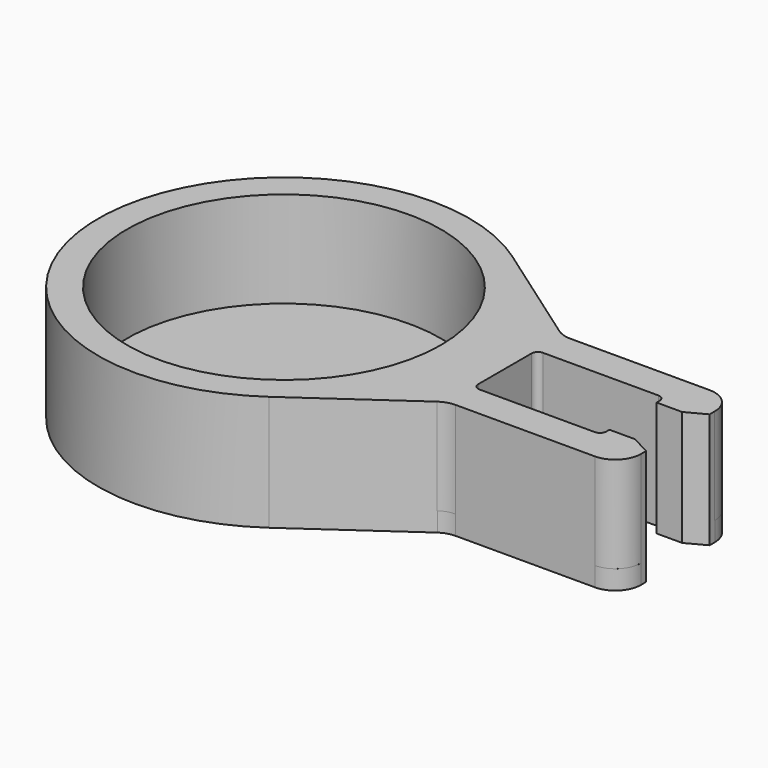
from build123d import *

# Parameters (mm, degrees)
F0_R        = 31.115
F1_DEPTH    = 19.05
F2_R        = 1.27
F3_R        = 5.08
F4_DEPTH    = 3.81
F5_T1_DEPTH = 6.9847500098
F6_T1_DEPTH = 7.826096392
F6_T3_DEPTH = 29.2095000049


# Not quite as in the source:
# - a fillet or chamfer that OpenCascade refuses, or shapes differently, is made with other operations: its cross-section is extruded or revolved along the edge and cut away or added


with BuildPart() as f1:
    # F0 (on Top) → F1 (new body)
    with BuildSketch(Plane.XY):
        with BuildLine():
            ThreePointArc((-22.6388816051, -22.2593853014), (-11.1319360334, -9.104404806), (-6.985, 7.874))
            ThreePointArc((-6.985, 7.874), (-11.1319360334, 24.852404806), (-22.6388816051, 38.0073853014))
            ThreePointArc((-22.6388816051, 38.0073853014), (-80.645, 7.874), (-22.6388816051, -22.2593853014))
        make_face()
        with Locations((-43.815, 7.874)):
            Circle(F0_R, mode=Mode.SUBTRACT)
        with BuildLine():
            Line((-6.985, 7.874), (0, 7.874))
            Line((0, 7.874), (0, 15.748))
            Line((0, 15.748), (25.4, 15.748))
            Line((25.4, 15.748), (34.29, 15.748))
            Line((34.29, 15.748), (34.29, 22.098))
            Line((34.29, 22.098), (0, 22.098))
            Line((0, 22.098), (-22.6388816051, 38.0073853014))
            ThreePointArc((-22.6388816051, 38.0073853014), (-11.1319360334, 24.852404806), (-6.985, 7.874))
        make_face()
        with BuildLine():
            Line((25.4, 0), (0, 0))
            Line((0, 0), (0, 7.874))
            Line((0, 7.874), (-6.985, 7.874))
            ThreePointArc((-6.985, 7.874), (-11.1319360334, -9.104404806), (-22.6388816051, -22.2593853014))
            Line((-22.6388816051, -22.2593853014), (0, -6.35))
            Line((0, -6.35), (34.29, -6.35))
            Line((34.29, -6.35), (34.29, 0))
            Line((34.29, 0), (25.4, 0))
        make_face()
        Polygon((25.4, 2.032), (25.4, 0), (34.29, 0), (30.48, 2.032), align=None)
        Polygon((34.29, 15.748), (25.4, 15.748), (25.4, 13.716), (30.48, 13.716), align=None)
    extrude(amount=F1_DEPTH)

    # F2
    f2_edges = [f1.edges().sort_by_distance(p)[0] for p in [
        (0, 15.748, 9.525),
        (25.4, 15.748, 9.525),
        (0, 0, 9.525),
        (25.4, 0, 9.525),
    ]]
    fillet(f2_edges, radius=F2_R)

    # F3
    f3_edges = [f1.edges().sort_by_distance(p)[0] for p in [
        (34.29, -6.35, 9.525),
        (34.29, 22.098, 9.525),
        (0, -6.35, 9.525),
        (0, 22.098, 9.525),
    ]]
    fillet(f3_edges, radius=F3_R)

    # F0 (on Top) → F4 (join)
    with BuildSketch(Plane.XY):
        with BuildLine():
            ThreePointArc((-22.6388816051, -22.2593853014), (-11.1319360334, -9.104404806), (-6.985, 7.874))
            ThreePointArc((-6.985, 7.874), (-11.1319360334, 24.852404806), (-22.6388816051, 38.0073853014))
            ThreePointArc((-22.6388816051, 38.0073853014), (-80.645, 7.874), (-22.6388816051, -22.2593853014))
        make_face()
        with Locations((-43.815, 7.874)):
            Circle(F0_R, mode=Mode.SUBTRACT)
        with Locations((-43.815, 7.874)):
            Circle(F0_R)
        with BuildLine():
            Line((25.4, 0), (0, 0))
            Line((0, 0), (0, 7.874))
            Line((0, 7.874), (-6.985, 7.874))
            ThreePointArc((-6.985, 7.874), (-11.1319360334, -9.104404806), (-22.6388816051, -22.2593853014))
            Line((-22.6388816051, -22.2593853014), (0, -6.35))
            Line((0, -6.35), (34.29, -6.35))
            Line((34.29, -6.35), (34.29, 0))
            Line((34.29, 0), (25.4, 0))
        make_face()
        with BuildLine():
            Line((-6.985, 7.874), (0, 7.874))
            Line((0, 7.874), (0, 15.748))
            Line((0, 15.748), (25.4, 15.748))
            Line((25.4, 15.748), (34.29, 15.748))
            Line((34.29, 15.748), (34.29, 22.098))
            Line((34.29, 22.098), (0, 22.098))
            Line((0, 22.098), (-22.6388816051, 38.0073853014))
            ThreePointArc((-22.6388816051, 38.0073853014), (-11.1319360334, 24.852404806), (-6.985, 7.874))
        make_face()
        Polygon((34.29, 15.748), (25.4, 15.748), (25.4, 13.716), (30.48, 13.716), align=None)
        Polygon((25.4, 2.032), (25.4, 0), (34.29, 0), (30.48, 2.032), align=None)
    extrude(amount=-F4_DEPTH)

    # F5: fillet of radius 1.27 on 4 edges, made by hand

    # F5_s2 → F5_t1 (join)
    with BuildSketch(Plane.XY.offset(-3.81)):
        with BuildLine():
            ThreePointArc((24.1301, -0.0001), (25.0281256121, 0.3718743879), (25.4001, 1.2699))
            Line((25.4001, 1.2699), (25.4255, 1.2699))
            ThreePointArc((25.4255, 1.2699), (25.4254, 0.63495), (25.4254, 0))
            Line((25.4254, 0), (25.4, -0.0254))
            ThreePointArc((25.4, -0.0254), (24.76505, -0.0254), (24.1301, -0.0255))
            Line((24.1301, -0.0255), (24.1301, -0.0001))
        make_face()
        with BuildLine():
            ThreePointArc((25.4001, 14.4781), (25.0281256121, 15.3761256121), (24.1301, 15.7481))
            Line((24.1301, 15.7481), (24.1301, 15.7735))
            ThreePointArc((24.1301, 15.7735), (24.76505, 15.7734), (25.4, 15.7734))
            Line((25.4, 15.7734), (25.4254, 15.748))
            ThreePointArc((25.4254, 15.748), (25.4254, 15.11305), (25.4255, 14.4781))
            Line((25.4255, 14.4781), (25.4001, 14.4781))
        make_face()
        with BuildLine():
            ThreePointArc((1.2699, 15.7481), (0.3718743879, 15.3761256121), (-0.0001, 14.4781))
            Line((-0.0001, 14.4781), (-0.0255, 14.4781))
            ThreePointArc((-0.0255, 14.4781), (-0.0254, 15.11305), (-0.0254, 15.748))
            Line((-0.0254, 15.748), (0, 15.7734))
            ThreePointArc((0, 15.7734), (0.63495, 15.7734), (1.2699, 15.7735))
            Line((1.2699, 15.7735), (1.2699, 15.7481))
        make_face()
        with BuildLine():
            ThreePointArc((-0.0001, 1.2699), (0.3718743879, 0.3718743879), (1.2699, -0.0001))
            Line((1.2699, -0.0001), (1.2699, -0.0255))
            ThreePointArc((1.2699, -0.0255), (0.63495, -0.0254), (0, -0.0254))
            Line((0, -0.0254), (-0.0254, 0))
            ThreePointArc((-0.0254, 0), (-0.0254, 0.63495), (-0.0255, 1.2699))
            Line((-0.0255, 1.2699), (-0.0001, 1.2699))
        make_face()
    extrude(amount=F5_T1_DEPTH)

    # F6: fillet of radius 5.08 on 4 edges, made by hand

    # F6_s2 → F6_t1 (join)
    with BuildSketch(Plane.XY.offset(-3.81)):
        with BuildLine():
            ThreePointArc((-1.3144053628, -7.2735709929), (0.0747322104, -6.5863191265), (1.6064385537, -6.3499))
            Line((1.6064385537, -6.3499), (1.6064385537, -6.2483))
            ThreePointArc((1.6064385537, -6.2483), (0.8032192768, -6.2484), (0, -6.2484))
            Line((0, -6.2484), (-0.0584168783, -6.2668734199))
            ThreePointArc((-0.0584168783, -6.2668734199), (-0.7155908113, -6.7286998251), (-1.3728222412, -7.1904444128))
            Line((-1.3728222412, -7.1904444128), (-1.3144053628, -7.2735709929))
        make_face()
        with BuildLine():
            ThreePointArc((-1.3144053628, 23.0215709929), (0.0747322104, 22.3343191265), (1.6064385537, 22.0979))
            Line((1.6064385537, 22.0979), (1.6064385537, 21.9963))
            ThreePointArc((1.6064385537, 21.9963), (0.8032192768, 21.9964), (0, 21.9964))
            Line((0, 21.9964), (-0.0584168783, 22.0148734199))
            ThreePointArc((-0.0584168783, 22.0148734199), (-0.7155908113, 22.4766998251), (-1.3728222412, 22.9384444128))
            Line((-1.3728222412, 22.9384444128), (-1.3144053628, 23.0215709929))
        make_face()
    extrude(amount=F6_T1_DEPTH)

    # F6_s4 → F6_t3 (cut)
    with BuildSketch(Plane.XY.offset(-16.5097500025)):
        with BuildLine():
            ThreePointArc((29.2101, -6.3501), (32.8022024484, -4.8622024484), (34.2901, -1.2701))
            Line((34.2901, -1.2701), (34.3917, -1.2701))
            ThreePointArc((34.3917, -1.2701), (34.3916, -3.81005), (34.3916, -6.35))
            Line((34.3916, -6.35), (34.29, -6.4516))
            ThreePointArc((34.29, -6.4516), (31.75005, -6.4516), (29.2101, -6.4517))
            Line((29.2101, -6.4517), (29.2101, -6.3501))
        make_face()
        with BuildLine():
            ThreePointArc((29.2101, 22.0981), (32.8022024484, 20.6102024484), (34.2901, 17.0181))
            Line((34.2901, 17.0181), (34.3917, 17.0181))
            ThreePointArc((34.3917, 17.0181), (34.3916, 19.55805), (34.3916, 22.098))
            Line((34.3916, 22.098), (34.29, 22.1996))
            ThreePointArc((34.29, 22.1996), (31.75005, 22.1996), (29.2101, 22.1997))
            Line((29.2101, 22.1997), (29.2101, 22.0981))
        make_face()
    extrude(amount=F6_T3_DEPTH, mode=Mode.SUBTRACT)


solid = f1.part
